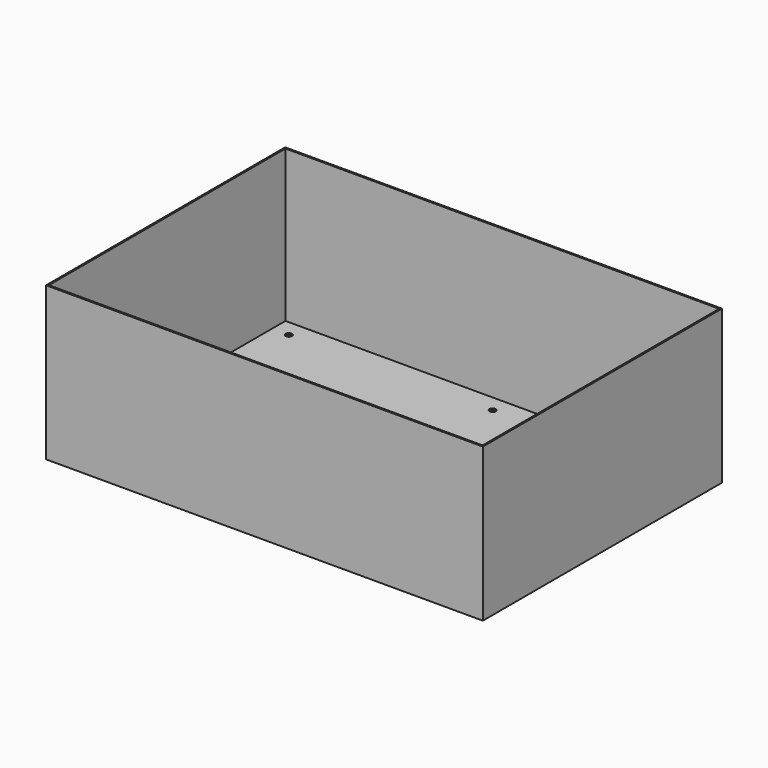
from build123d import *

# Parameters (mm, degrees)
F0_W     = 285
F0_H     = 195
F1_DEPTH = 100
F2_T     = -1
F3_D     = 4.1


# Not quite as in the source:
# - a feature names something its author has since deleted; it is built from what else it names


with BuildPart() as f1:
    # F0 (on Top) → F1 (new body)
    with BuildSketch(Plane.XY):
        with Locations((12.5, 2.5)):
            Rectangle(F0_W, F0_H)
    extrude(amount=F1_DEPTH)

    # F2
    f2_openings = [f1.faces().sort_by_distance(p)[0] for p in [
        (12.5, 2.5, 100),
    ]]
    offset(amount=F2_T, openings=f2_openings)

    # F3 (through all)
    with Locations(Plane(origin=(0, 0, 0), x_dir=(1, 0, 0), z_dir=(0, 0, -1))):
        with Locations((15, -88), (-118, -88), (143, 83), (-118, 83)):
            Hole(F3_D / 2)


solid = f1.part
